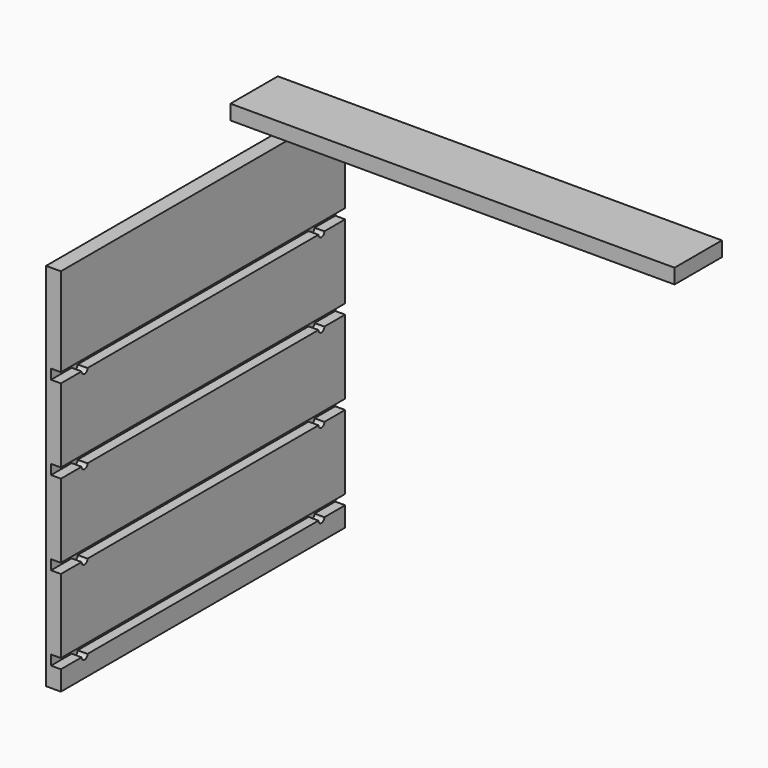
from build123d import *

# Parameters (mm, degrees)
F0_W     = 457.2
F0_H     = 476.25
F2_DEPTH = 19.05
F3_DEPTH = 12.7
F4_DEPTH = 12.7
F5_W     = 76.2
F5_H     = 19.05
F6_DEPTH = 571.5


# Not quite as in the source:
# - a feature names something its author has since deleted; it is built from what else it names


with BuildPart() as f2:
    # F0 (on Right) → F2 (new body)
    with BuildSketch(Plane.YZ):
        with Locations((-166.1135266319, -210.7972649872)):
            Rectangle(F0_W, F0_H)
    extrude(amount=-F2_DEPTH)

    # F1 (on face) → F3 (cut)
    with BuildSketch(Plane.YZ):
        with BuildLine():
            Line((-394.7135266319, -410.8222649872), (-394.7135266319, -423.5222649872))
            Line((-394.7135266319, -423.5222649872), (-361.3760266319, -423.5222649872))
            ThreePointArc((-361.3760266319, -423.5222649872), (-356.6135266319, -428.2847649872), (-351.8510266319, -423.5222649872))
            Line((-351.8510266319, -423.5222649872), (19.6239733681, -423.5222649872))
            ThreePointArc((19.6239733681, -423.5222649872), (24.3864733681, -428.2847649872), (29.1489733681, -423.5222649872))
            Line((29.1489733681, -423.5222649872), (62.4864733681, -423.5222649872))
            Line((62.4864733681, -423.5222649872), (62.4864733681, -410.8222649872))
            Line((62.4864733681, -410.8222649872), (-394.7135266319, -410.8222649872))
        make_face()
    extrude(amount=-F3_DEPTH, mode=Mode.SUBTRACT)

    # F1 (on face) → F4 (cut)
    with BuildSketch(Plane.YZ):
        with BuildLine():
            Line((-394.7135266319, -302.8722649872), (-394.7135266319, -315.5722649872))
            Line((-394.7135266319, -315.5722649872), (-361.3760266319, -315.5722649872))
            ThreePointArc((-361.3760266319, -315.5722649872), (-356.6135266319, -320.3347649872), (-351.8510266319, -315.5722649872))
            Line((-351.8510266319, -315.5722649872), (19.6239733681, -315.5722649872))
            ThreePointArc((19.6239733681, -315.5722649872), (24.3864733681, -320.3347649872), (29.1489733681, -315.5722649872))
            Line((29.1489733681, -315.5722649872), (62.4864733681, -315.5722649872))
            Line((62.4864733681, -315.5722649872), (62.4864733681, -302.8722649872))
            Line((62.4864733681, -302.8722649872), (-394.7135266319, -302.8722649872))
        make_face()
        with BuildLine():
            Line((-394.7135266319, -194.9222649872), (-394.7135266319, -207.6222649872))
            Line((-394.7135266319, -207.6222649872), (-361.3760266319, -207.6222649872))
            ThreePointArc((-361.3760266319, -207.6222649872), (-356.6135266319, -212.3847649872), (-351.8510266319, -207.6222649872))
            Line((-351.8510266319, -207.6222649872), (19.6239733681, -207.6222649872))
            ThreePointArc((19.6239733681, -207.6222649872), (24.3864733681, -212.3847649872), (29.1489733681, -207.6222649872))
            Line((29.1489733681, -207.6222649872), (62.4864733681, -207.6222649872))
            Line((62.4864733681, -207.6222649872), (62.4864733681, -194.9222649872))
            Line((62.4864733681, -194.9222649872), (-394.7135266319, -194.9222649872))
        make_face()
        with BuildLine():
            Line((-394.7135266319, -86.9722649872), (-394.7135266319, -99.6722649872))
            Line((-394.7135266319, -99.6722649872), (-361.3760266319, -99.6722649872))
            ThreePointArc((-361.3760266319, -99.6722649872), (-356.6135266319, -104.4347649872), (-351.8510266319, -99.6722649872))
            Line((-351.8510266319, -99.6722649872), (19.6239733681, -99.6722649872))
            ThreePointArc((19.6239733681, -99.6722649872), (24.3864733681, -104.4347649872), (29.1489733681, -99.6722649872))
            Line((29.1489733681, -99.6722649872), (62.4864733681, -99.6722649872))
            Line((62.4864733681, -99.6722649872), (62.4864733681, -86.9722649872))
            Line((62.4864733681, -86.9722649872), (-394.7135266319, -86.9722649872))
        make_face()
    extrude(amount=-F4_DEPTH, mode=Mode.SUBTRACT)


with BuildPart() as f6:
    # F5 (on Right) → F6 (new body)
    with BuildSketch(Plane.YZ):
        with Locations((-83.9446932077, 96.8780869972)):
            Rectangle(F5_W, F5_H)
    extrude(amount=F6_DEPTH)


solid = Compound([f2.part, f6.part])
